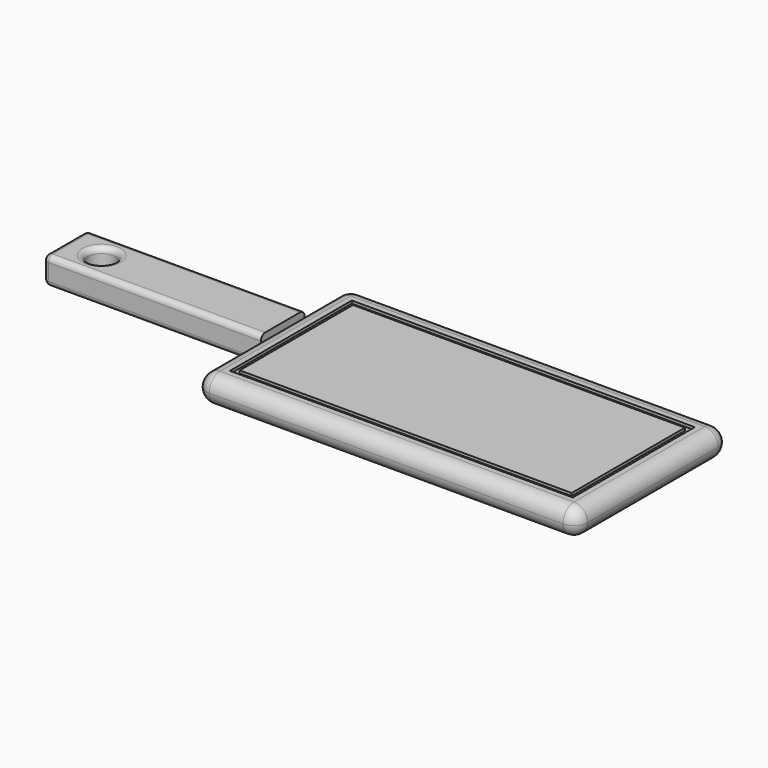
from build123d import *

# Parameters (mm, degrees)
F0_W     = 355.6
F0_H     = 177.8
F1_DEPTH = 25.4
F2_W     = 203.2
F2_H     = 50.8
F3_DEPTH = 25.4
F4_R     = 12.7
F5_DEPTH = 25.401
F6_R     = 5.08
F7_R     = 12.69999
F8_W     = 320.04
F8_H     = 142.24
F8_W_2   = 309.88
F8_H_2   = 132.08
F9_DEPTH = 2.54


# Not quite as in the source:
# - a fillet or chamfer is up to 0.001 mm smaller than in the source, because OpenCascade refuses the exact size


with BuildPart() as f1:
    # F0 (on Top) → F1 (new body)
    with BuildSketch(Plane.XY):
        with Locations((177.8, 88.9)):
            Rectangle(F0_W, F0_H)
    extrude(amount=F1_DEPTH)

    # F7 (radius 12.7 in the source; OpenCascade refuses exactly that, so slightly less here)
    f7_edges = [f1.edges().sort_by_distance(p)[0] for p in [
        (0, 88.9, 25.4),
        (0, 88.9, 0),
        (0, 177.8, 12.7),
        (177.8, 177.8, 25.4),
        (355.6, 177.8, 12.7),
        (355.6, 88.9, 0),
        (355.6, 88.9, 25.4),
        (0, 0, 12.7),
        (355.6, 0, 12.7),
        (177.8, 0, 0),
        (177.8, 0, 25.4),
        (177.8, 177.8, 0),
    ]]
    fillet(f7_edges, radius=F7_R)

    # F8 (on face) → F9 (cut)
    with BuildSketch(Plane.XY.offset(25.4)):
        with Locations((177.8, 88.9)):
            Rectangle(F8_W, F8_H)
        with Locations((177.8, 88.9)):
            Rectangle(F8_W_2, F8_H_2, mode=Mode.SUBTRACT)
    extrude(amount=-F9_DEPTH, mode=Mode.SUBTRACT)


with BuildPart() as f3:
    # F2 (on face) → F3 (new body)
    with BuildSketch(Plane.XY.offset(25.4)):
        with Locations((-101.6, 101.6)):
            Rectangle(F2_W, F2_H)
    extrude(amount=-F3_DEPTH)

    # F4 (on face) → F5 (cut, through all)
    with BuildSketch(Plane.XY.offset(25.4)):
        with Locations((-169.0784096718, 101.6)):
            Circle(F4_R)
    extrude(amount=-F5_DEPTH, mode=Mode.SUBTRACT)

    # F6
    f6_edges = [f3.edges().sort_by_distance(p)[0] for p in [
        (-181.77841, 101.6, 25.4),
        (-181.77841, 101.6, 0),
        (-101.6, 76.2, 0),
        (-203.2, 76.2, 12.7),
        (-203.2, 101.6, 0),
        (-203.2, 101.6, 25.4),
        (-101.6, 127, 25.4),
        (-203.2, 127, 12.7),
        (-101.6, 127, 0),
        (-101.6, 76.2, 25.4),
    ]]
    fillet(f6_edges, radius=F6_R)


solid = Compound([f1.part, f3.part])
